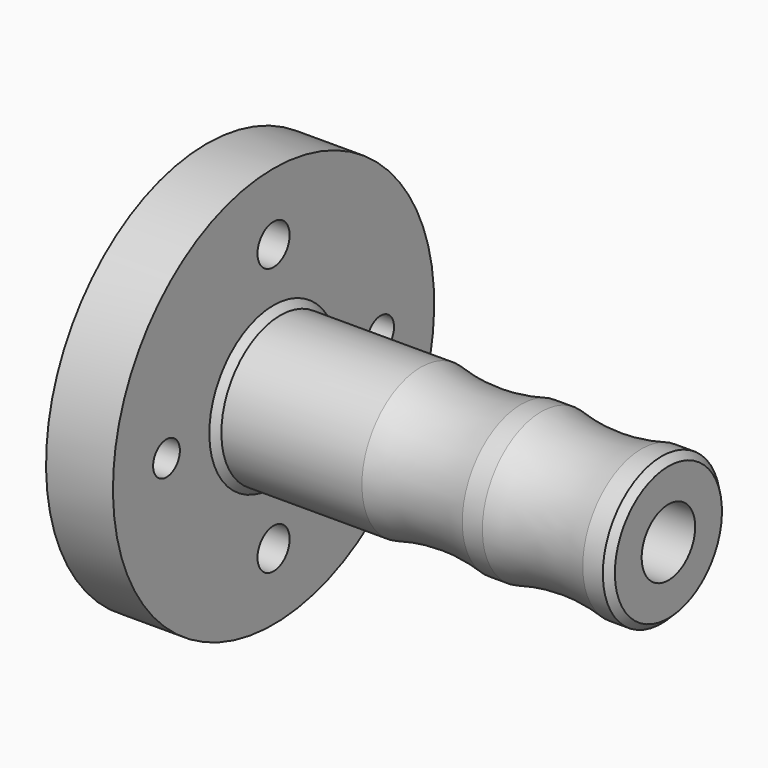
from build123d import *

# Parameters (mm, degrees)
F3_D     = 6
F5_D     = 5
F7_D     = 10
F7_DEPTH = 20
F7_TIP   = 3.0043030951


# Not quite as in the source:
# - a pattern or mirror of a feature is missing from the dataset's text; its kind, count and spacing are read off the source's solid


with BuildPart() as f1:
    # F0 (on Front) → F1 (revolve)
    with BuildSketch(Plane.XZ):
        with BuildLine():
            Line((-58, 11), (-59, 12))
            Line((-59, 12), (-59, 30))
            Line((-59, 30), (-69, 30))
            Line((-69, 30), (-69, 0))
            Line((-69, 0), (0, 0))
            Line((0, 0), (0, 10))
            Line((0, 10), (-1, 11))
            Line((-1, 11), (-4, 11))
            ThreePointArc((-4, 11), (-11.5, 10.0473750966), (-19, 11))
            Line((-19, 11), (-22, 11))
            ThreePointArc((-22, 11), (-29.5, 10.0473750966), (-37, 11))
            Line((-37, 11), (-58, 11))
        make_face()
    revolve(axis=Axis((-18.6788269784, 0, 0), (1, 0, 0)))

    # F3 (through all)
    with Locations(Plane(origin=(-69, 0, 0), x_dir=(0, -1, 0), z_dir=(-1, 0, 0))):
        with Locations((0, 20)):
            f3 = Hole(F3_D / 2)

    # F3_copies: F3 across plane
    add(f3.mirror(Plane(origin=(0, 0, 0), x_dir=(-1, 0, 0), z_dir=(0, 0, -1))), mode=Mode.SUBTRACT)

    # F5 (through all)
    with Locations(Plane(origin=(-69, 0, 0), x_dir=(0, -1, 0), z_dir=(-1, 0, 0))):
        with Locations((20, 0)):
            f5 = Hole(F5_D / 2)

    # F5_copies: F5 across plane
    add(f5.mirror(Plane.ZX), mode=Mode.SUBTRACT)

    # F7
    with Locations(Plane.YZ):
        with Locations((0, 0)):
            Hole(F7_D / 2, depth=F7_DEPTH)
            with Locations((0, 0, -(F7_DEPTH + F7_TIP / 2))):  # 118° drill point
                Cone(0, F7_D / 2, F7_TIP, mode=Mode.SUBTRACT)


solid = f1.part
